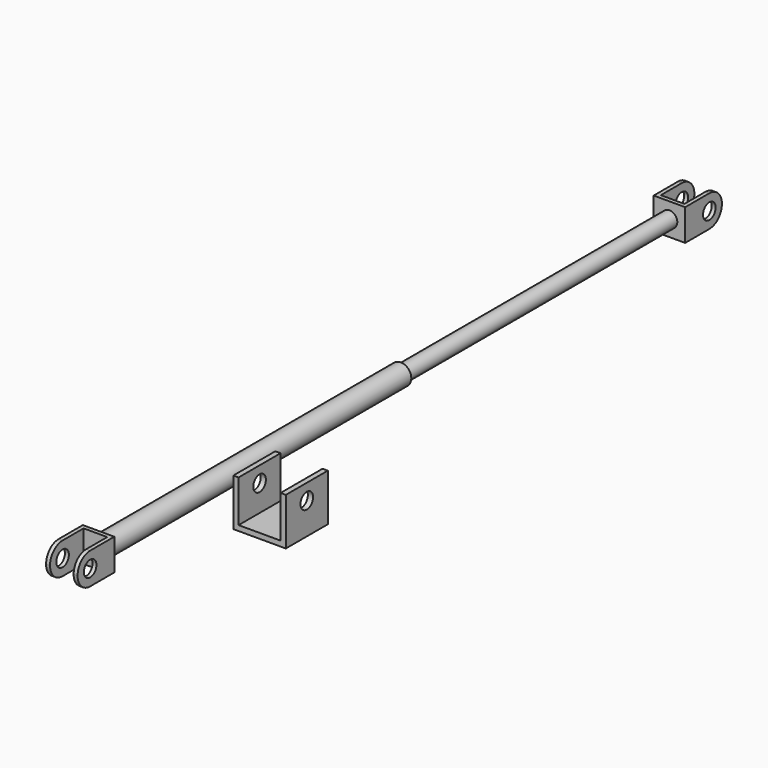
from build123d import *

# Parameters (mm, degrees)
F0_W      = 50.8
F0_H      = 38.1
F0_R      = 9.525
F1_DEPTH  = 4.7625
F2_R      = 19.04999
F3_W      = 33.3375
F3_H      = 38.1
F3_W_2    = 4.7625
F4_DEPTH  = 4.7625
F5_W      = 50.8
F5_H      = 38.1
F5_R      = 9.525
F6_DEPTH  = 4.7625
F7_R      = 19.04999
F8_R      = 12.7
F9_DEPTH  = 457.2
F11_D     = 19.05
F11_DEPTH = 457.2
F11_TIP   = 5.7231973962
F12_R     = 9.525
F13_DEPTH = 406.4
F14_W     = 38.1
F14_H     = 38.1
F14_R     = 9.525
F15_DEPTH = 4.7625
F16_W     = 50.8
F16_H     = 38.1
F16_R     = 9.525
F17_DEPTH = 4.7625
F18_R     = 19.04999
F19_W     = 50.8
F19_H     = 38.1
F19_R     = 9.525
F20_DEPTH = 4.7625
F21_R     = 19.04999
F22_W     = 63.5
F22_H     = 63.5
F23_DEPTH = 6.35
F24_W     = 63.5
F24_H     = 50.8
F24_R     = 9.525
F25_DEPTH = 6.35
F26_W     = 63.5
F26_H     = 50.8
F26_R     = 9.525
F27_DEPTH = 6.35


# Not quite as in the source:
# - a fillet or chamfer is up to 0.001 mm smaller than in the source, because OpenCascade refuses the exact size


with BuildPart() as f1:
    # F0 (on Right) → F1 (new body)
    with BuildSketch(Plane.YZ):
        with Locations((-148.0474919081, 9.8244957626)):
            Rectangle(F0_W, F0_H)
        with Locations((-154.3974919081, 9.8244957626)):
            Circle(F0_R, mode=Mode.SUBTRACT)
    extrude(amount=F1_DEPTH)

    # F2 (radius 19.05 in the source; OpenCascade refuses exactly that, so slightly less here)
    f2_edges = [f1.edges().sort_by_distance(p)[0] for p in [
        (2.38125, -173.447492, 28.874496),
        (2.38125, -173.447492, -9.225504),
    ]]
    fillet(f2_edges, radius=F2_R)

    # F3 (on face) → F4 (join)
    with BuildSketch(Plane(origin=(0, -122.6474919081, 0), x_dir=(-1, 0, 0), z_dir=(0, 1, 0))):
        with Locations((16.66875, 9.8244957626)):
            Rectangle(F3_W, F3_H)
        with Locations((-2.38125, 9.8244957626)):
            Rectangle(F3_W_2, F3_H)
    extrude(amount=F4_DEPTH)

    # F5 (on face) → F6 (join)
    with BuildSketch(Plane(origin=(-33.3375, 0, 0), x_dir=(0, -1, 0), z_dir=(-1, 0, 0))):
        with Locations((148.0474919081, 9.8244957626)):
            Rectangle(F5_W, F5_H)
        with Locations((154.4447690248, 9.8060360178)):
            Circle(F5_R, mode=Mode.SUBTRACT)
    extrude(amount=-F6_DEPTH)

    # F7 (radius 19.05 in the source; OpenCascade refuses exactly that, so slightly less here)
    f7_edges = [f1.edges().sort_by_distance(p)[0] for p in [
        (-30.95625, -173.447492, 28.874496),
        (-30.95625, -173.447492, -9.225504),
    ]]
    fillet(f7_edges, radius=F7_R)

    # F8 (on face) → F9 (join)
    with BuildSketch(Plane(origin=(0, -117.8849919081, 0), x_dir=(-1, 0, 0), z_dir=(0, 1, 0))):
        with Locations((14.2875, 9.8244957626)):
            Circle(F8_R)
    extrude(amount=F9_DEPTH)

    # F11
    with Locations(Plane(origin=(0, 339.3150080919, 0), x_dir=(-1, 0, 0), z_dir=(0, 1, 0))):
        with Locations((14.2875, 9.8244957626)):
            Hole(F11_D / 2, depth=F11_DEPTH)
            with Locations((0, 0, -(F11_DEPTH + F11_TIP / 2))):  # 118° drill point
                Cone(0, F11_D / 2, F11_TIP, mode=Mode.SUBTRACT)


with BuildPart() as f13:
    # F12 (on face) → F13 (new body)
    with BuildSketch(Plane(origin=(0, 339.3150080919, 0), x_dir=(-1, 0, 0), z_dir=(0, 1, 0))):
        with Locations((14.2875, 9.8244957626)):
            Circle(F12_R)
    extrude(amount=F13_DEPTH)

    # F14 (on face) → F15 (join)
    with BuildSketch(Plane(origin=(0, 745.7150080919, 0), x_dir=(-1, 0, 0), z_dir=(0, 1, 0))):
        with Locations((14.2927456155, 9.8272960141)):
            Rectangle(F14_W, F14_H)
        with Locations((14.2875, 9.8244957626)):
            Circle(F14_R, mode=Mode.SUBTRACT)
        with Locations((14.2875, 9.8244957626)):
            Circle(F14_R)
    extrude(amount=F15_DEPTH)

    # F16 (on face) → F17 (join)
    with BuildSketch(Plane.YZ.offset(4.7572543845)):
        with Locations((775.8775080919, 9.8272960141)):
            Rectangle(F16_W, F16_H)
        with Locations((782.2275080919, 9.8272960141)):
            Circle(F16_R, mode=Mode.SUBTRACT)
    extrude(amount=-F17_DEPTH)

    # F18 (radius 19.05 in the source; OpenCascade refuses exactly that, so slightly less here)
    f18_edges = [f13.edges().sort_by_distance(p)[0] for p in [
        (2.376004, 801.277508, 28.877296),
        (2.376004, 801.277508, -9.222704),
    ]]
    fillet(f18_edges, radius=F18_R)

    # F19 (on face) → F20 (join)
    with BuildSketch(Plane(origin=(-33.3427456155, 0, 0), x_dir=(0, -1, 0), z_dir=(-1, 0, 0))):
        with Locations((-775.8775080919, 9.8272960141)):
            Rectangle(F19_W, F19_H)
        with Locations((-782.2275080919, 9.8272960141)):
            Circle(F19_R, mode=Mode.SUBTRACT)
    extrude(amount=-F20_DEPTH)

    # F21 (radius 19.05 in the source; OpenCascade refuses exactly that, so slightly less here)
    f21_edges = [f13.edges().sort_by_distance(p)[0] for p in [
        (-30.961496, 801.277508, 28.877296),
        (-30.961496, 801.277508, -9.222704),
    ]]
    fillet(f21_edges, radius=F21_R)


with BuildPart() as f23:
    # F22 (on Top) → F23 (new body)
    with BuildSketch(Plane.XY):
        with Locations((80.0405043066, 39.5346571803)):
            Rectangle(F22_W, F22_H)
    extrude(amount=F23_DEPTH)

    # F24 (on face) → F25 (join)
    with BuildSketch(Plane.YZ.offset(111.7905043066)):
        with Locations((39.5346571803, 31.75)):
            Rectangle(F24_W, F24_H)
        with Locations((39.5346571803, 38.1)):
            Circle(F24_R, mode=Mode.SUBTRACT)
    extrude(amount=-F25_DEPTH)

    # F26 (on face) → F27 (join)
    with BuildSketch(Plane(origin=(48.2905043066, 0, 0), x_dir=(0, -1, 0), z_dir=(-1, 0, 0))):
        with Locations((-39.5346571803, 31.75)):
            Rectangle(F26_W, F26_H)
        with Locations((-39.5346571803, 38.1)):
            Circle(F26_R, mode=Mode.SUBTRACT)
    extrude(amount=-F27_DEPTH)


solid = Compound([f1.part, f13.part, f23.part])
